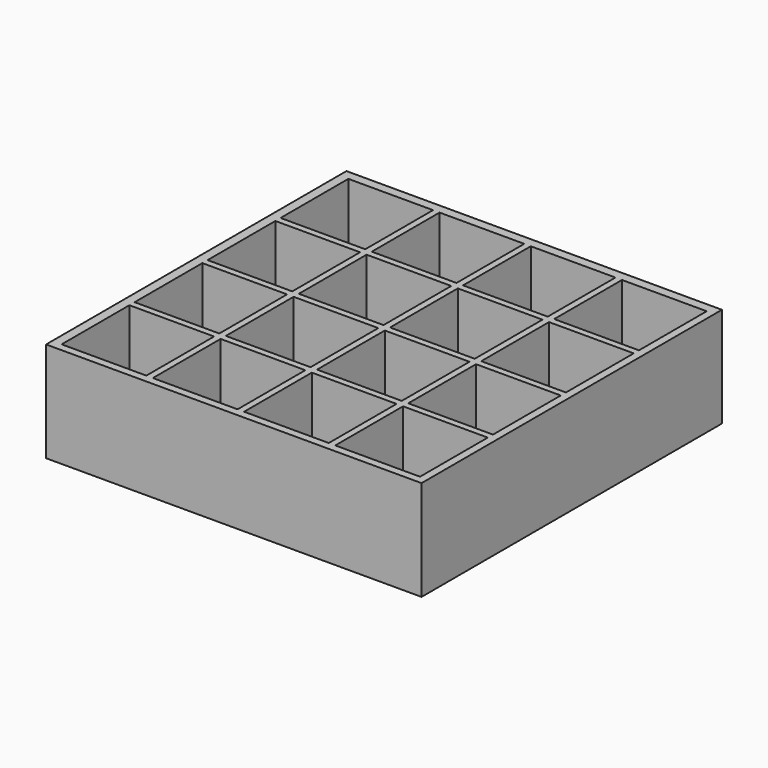
from build123d import *

# Parameters (mm, degrees)
F0_W     = 1463.675
F0_H     = 1463.675
F0_W_2   = 330.2
F0_H_2   = 330.2
F1_DEPTH = 390.525
F2_SCALE = 0.05


with BuildPart() as f1:
    # F0 (on Top) → F1 (new body)
    with BuildSketch(Plane.XY):
        Rectangle(F0_W, F0_H)
        with Locations((-530.225, -536.575)):
            Rectangle(F0_W_2, F0_H_2, mode=Mode.SUBTRACT)
        with Locations((-174.625, -536.575)):
            Rectangle(F0_W_2, F0_H_2, mode=Mode.SUBTRACT)
        with Locations((-530.225, -180.975)):
            Rectangle(F0_W_2, F0_H_2, mode=Mode.SUBTRACT)
        with Locations((-174.625, -180.975)):
            Rectangle(F0_W_2, F0_H_2, mode=Mode.SUBTRACT)
        with Locations((180.975, -536.575)):
            Rectangle(F0_W_2, F0_H_2, mode=Mode.SUBTRACT)
        with Locations((536.575, -536.575)):
            Rectangle(F0_W_2, F0_H_2, mode=Mode.SUBTRACT)
        with Locations((180.975, -180.975)):
            Rectangle(F0_W_2, F0_H_2, mode=Mode.SUBTRACT)
        with Locations((536.575, -180.975)):
            Rectangle(F0_W_2, F0_H_2, mode=Mode.SUBTRACT)
        with Locations((-530.225, 174.625)):
            Rectangle(F0_W_2, F0_H_2, mode=Mode.SUBTRACT)
        with Locations((-174.625, 174.625)):
            Rectangle(F0_W_2, F0_H_2, mode=Mode.SUBTRACT)
        with Locations((-530.225, 530.225)):
            Rectangle(F0_W_2, F0_H_2, mode=Mode.SUBTRACT)
        with Locations((-174.625, 530.225)):
            Rectangle(F0_W_2, F0_H_2, mode=Mode.SUBTRACT)
        with Locations((180.975, 174.625)):
            Rectangle(F0_W_2, F0_H_2, mode=Mode.SUBTRACT)
        with Locations((536.575, 174.625)):
            Rectangle(F0_W_2, F0_H_2, mode=Mode.SUBTRACT)
        with Locations((180.975, 530.225)):
            Rectangle(F0_W_2, F0_H_2, mode=Mode.SUBTRACT)
        with Locations((536.575, 530.225)):
            Rectangle(F0_W_2, F0_H_2, mode=Mode.SUBTRACT)
    extrude(amount=F1_DEPTH)


with BuildPart() as f1_1:
    # F2: moved
    add(f1.part.scale(F2_SCALE))


solid = f1_1.part
